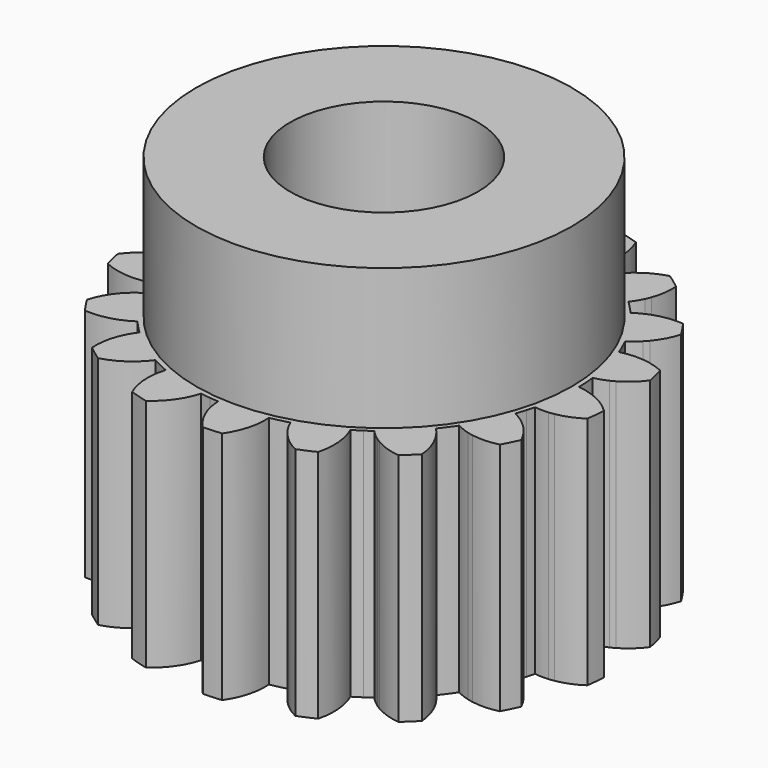
from build123d import *

# Parameters (mm, degrees)
F0_R     = 10
F1_DEPTH = 25
F2_COUNT = 18
F3_R     = 20
F3_R_2   = 10
F4_DEPTH = 15


with BuildPart() as f1:
    # F0 (on Top) → F1 (new body)
    with BuildSketch(Plane.XY):
        with BuildLine():
            ThreePointArc((7.9296197565, 23.5951858335), (6.9911317973, 23.8900761864), (6.0417249702, 24.1476546146))
            ThreePointArc((6.0417249702, 24.1476546146), (4.3226425573, 22.4330749308), (3.2648662162, 20.2476374354))
            ThreePointArc((3.2648662162, 20.2476374354), (5.7837443287, 19.6767495961), (8.2108987358, 18.7938105523))
            ThreePointArc((8.2108987358, 18.7938105523), (8.3954934616, 19.5156536929), (8.4994507341, 20.2534379554))
            ThreePointArc((8.4994507341, 20.2534379554), (8.5176465567, 20.5391701676), (8.5237154667, 20.8254168329))
            ThreePointArc((8.5237154667, 20.8254168329), (8.373521449, 22.2418004346), (7.9296197565, 23.5951858335))
        make_face()
        with BuildLine():
            ThreePointArc((4.0264902572, 14.4598933509), (-1.7431476836, 15.057566034), (-4.9211585336, 19.9100068261))
            ThreePointArc((-4.9211585336, 19.9100068261), (-12.6431262329, -16.1486077476), (20.5091729021, 0))
            ThreePointArc((20.5091729021, 0), (19.2415803806, 7.0984334598), (15.5954927821, 13.3194135761))
            ThreePointArc((15.5954927821, 13.3194135761), (9.5256046991, 10.9946956396), (4.0264902572, 14.4598933509))
        make_face()
        Circle(F0_R, mode=Mode.SUBTRACT)
        with BuildLine():
            ThreePointArc((3.2648662162, 20.2476374354), (-0.8451772993, 20.4917507417), (-4.9211585336, 19.9100068261))
            ThreePointArc((-4.9211585336, 19.9100068261), (-1.7431476836, 15.057566034), (4.0264902572, 14.4598933509))
            ThreePointArc((4.0264902572, 14.4598933509), (3.0384725246, 17.2738616412), (3.2648662162, 20.2476374354))
        make_face()
        with BuildLine():
            ThreePointArc((4.0264902572, 14.4598933509), (9.5256046991, 10.9946956396), (15.5954927821, 13.3194135761))
            ThreePointArc((15.5954927821, 13.3194135761), (12.2138579016, 16.4756744411), (8.2108987358, 18.7938105523))
            ThreePointArc((8.2108987358, 18.7938105523), (6.6287005247, 16.1344397874), (4.0264902572, 14.4598933509))
        make_face()
        with BuildLine():
            ThreePointArc((8.2108987358, 18.7938105523), (5.7837443287, 19.6767495961), (3.2648662162, 20.2476374354))
            ThreePointArc((3.2648662162, 20.2476374354), (3.0384725246, 17.2738616412), (4.0264902572, 14.4598933509))
            ThreePointArc((4.0264902572, 14.4598933509), (6.6287005247, 16.1344397874), (8.2108987358, 18.7938105523))
        make_face()
    extrude(amount=F1_DEPTH)

    # F2: F1 ×18 about axis
    f2_axis = Axis((0, 0, 25), (0, 0, 1))


with BuildPart() as f1_1:
    add(f1.part)
    for i in range(1, F2_COUNT):
        add(f1.part.rotate(f2_axis, i * 360 / F2_COUNT))

    # F3 (on face) → F4 (join)
    with BuildSketch(Plane.XY.offset(25)):
        Circle(F3_R)
        Circle(F3_R_2, mode=Mode.SUBTRACT)
    extrude(amount=F4_DEPTH)


solid = f1_1.part
